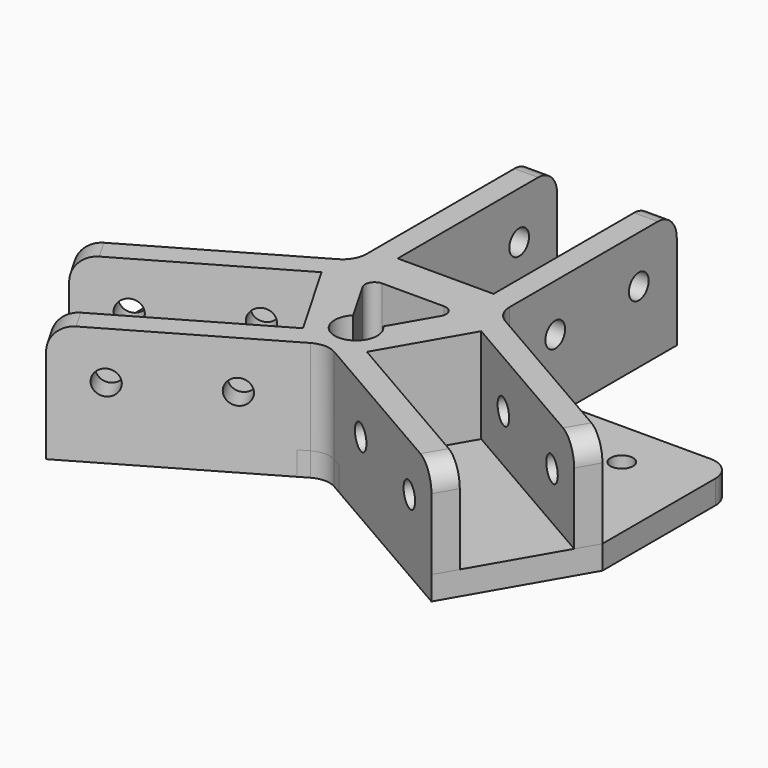
from build123d import *

# Parameters (mm, degrees)
F1_DEPTH    = 20
F2_R        = 2.6
F3_DEPTH    = 50.6016350946
F4_COUNT    = 3
F4_ANGLE    = 240
F6_DEPTH    = 5
F7_T1_DEPTH = 25
F10_DEPTH   = 5
F11_DEPTH   = 25.001
F12_R       = 2
F13_R       = 2.6
F13_R_2     = 2.372590354
F14_DEPTH   = 25.001
F15_R       = 5
F16_R       = 4.5
F17_DEPTH   = 20


# Not quite as in the source:
# - a fillet or chamfer that OpenCascade refuses, or shapes differently, is made with other operations: its cross-section is extruded or revolved along the edge and cut away or added


with BuildPart() as f1:
    # F0 (on Top) → F1 (new body)
    with BuildSketch(Plane.XY):
        Polygon((43.0992290895, -36.5458269543), (6.7261621305, -15.5458269543), (16.8261621305, 1.9478862021), (53.1992290895, -19.0521137979), (55.6992290895, -14.7219867789), (14.8979589003, 8.8346375481), (0, 0), (-0.2020410997, -17.3193296462), (40.5992290895, -40.8759539732), align=None)
    extrude(amount=F1_DEPTH)

    # F2 (on face) → F3 (cut, through all)
    with BuildSketch(Plane(origin=(-7.55, -13.0769835971, 0), x_dir=(0.8660254038, -0.5, 0), z_dir=(-0.5, -0.8660254038, 0))):
        with Locations((45.5979407522, 10)):
            Circle(F2_R)
        with Locations((23.5979407522, 10)):
            Circle(F2_R)
    extrude(amount=-F3_DEPTH, mode=Mode.SUBTRACT)

    # F4: F1 ×3 about axis
    f4_axis = Axis((0, 0, 10), (0, 0, -1))


with BuildPart() as f1_1:
    add(f1.part)
    for i in range(1, F4_COUNT):
        add(f1.part.rotate(f4_axis, i * F4_ANGLE / (F4_COUNT - 1)))

    # F5 (on face) → F6 (join)
    with BuildSketch(Plane(origin=(0, 0, 0), x_dir=(1, 0, 0), z_dir=(0, 0, -1))):
        Polygon((0, 17.4359781295), (-40.5992290895, 40.8759539732), (-55.6992290895, 14.7219867789), (-15.1, -8.7179890648), (-15.1, -55.5979407522), (15.1, -55.5979407522), (15.1, -8.7179890648), (55.6992290895, 14.7219867789), (40.5992290895, 40.8759539732), align=None)
    extrude(amount=F6_DEPTH)

    # F7: fillet of radius 5 on 3 edges, made by hand

    # F7_s2 → F7_t1 (join)
    with BuildSketch(Plane.XY.offset(-5)):
        with BuildLine():
            ThreePointArc((2.5, -18.8792383324), (0, -18.2093653514), (-2.5, -18.8792383324))
            Line((-2.5, -18.8792383324), (-2.55, -18.7926357921))
            ThreePointArc((-2.55, -18.7926357921), (-1.299975, -18.0710489919), (-0.05, -17.3493755891))
            Line((-0.05, -17.3493755891), (0.05, -17.3493755891))
            ThreePointArc((0.05, -17.3493755891), (1.299975, -18.0710489919), (2.55, -18.7926357921))
            Line((2.55, -18.7926357921), (2.5, -18.8792383324))
        make_face()
        with BuildLine():
            ThreePointArc((15.0999, 11.6046826757), (15.7697729811, 9.1046826757), (17.5999, 7.2745556568))
            Line((17.5999, 7.2745556568), (17.5499, 7.1879531164))
            ThreePointArc((17.5499, 7.1879531164), (16.299975, 7.9097131217), (15.05, 8.6313865244))
            Line((15.05, 8.6313865244), (15, 8.7179890648))
            ThreePointArc((15, 8.7179890648), (15, 10.1613358702), (14.9999, 11.6046826757))
            Line((14.9999, 11.6046826757), (15.0999, 11.6046826757))
        make_face()
        with BuildLine():
            ThreePointArc((-17.5999, 7.2745556568), (-15.7697729811, 9.1046826757), (-15.0999, 11.6046826757))
            Line((-15.0999, 11.6046826757), (-14.9999, 11.6046826757))
            ThreePointArc((-14.9999, 11.6046826757), (-15, 10.1613358702), (-15, 8.7179890648))
            Line((-15, 8.7179890648), (-15.05, 8.6313865244))
            ThreePointArc((-15.05, 8.6313865244), (-16.299975, 7.9097131217), (-17.5499, 7.1879531164))
            Line((-17.5499, 7.1879531164), (-17.5999, 7.2745556568))
        make_face()
    extrude(amount=F7_T1_DEPTH)

    # F9 (on face) → F10 (join)
    with BuildSketch(Plane(origin=(0, 0, -5), x_dir=(1, 0, 0), z_dir=(0, 0, -1))):
        with BuildLine():
            Line((-55.6992290895, 14.7219867789), (-55.6992290895, -20))
            Line((-55.6992290895, -20), (55.6992290895, -20))
            Line((55.6992290895, -20), (55.6992290895, 14.7219867789))
            Line((55.6992290895, 14.7219867789), (52.6519667355, 20))
            Line((52.6519667355, 20), (4.4410161514, 20))
            Line((4.4410161514, 20), (2.5, 18.8793538025))
            ThreePointArc((2.5, 18.8793538025), (0, 18.2094808214), (-2.5, 18.8793538025))
            Line((-2.5, 18.8793538025), (-4.4410161514, 20))
            Line((-4.4410161514, 20), (-52.6519667355, 20))
            Line((-52.6519667355, 20), (-55.6992290895, 14.7219867789))
        make_face()
    extrude(amount=-F10_DEPTH)

    # F8 (on face) → F11 (cut, through all)
    with BuildSketch(Plane.XY.offset(20)):
        Polygon((10, 5.0614941438), (-10, 5.0614941438), (0, -12.2590139319), align=None)
    extrude(amount=-F11_DEPTH, mode=Mode.SUBTRACT)

    # F12
    f12_edges = [f1_1.edges().sort_by_distance(p)[0] for p in [
        (10, 5.061494, 7.5),
        (-10, 5.061494, 7.5),
        (0, -12.259014, 7.5),
    ]]
    fillet(f12_edges, radius=F12_R)

    # F13 (on face) → F14 (cut, through all)
    with BuildSketch(Plane(origin=(0, 0, -5), x_dir=(1, 0, 0), z_dir=(0, 0, -1))):
        with Locations((-40, -10)):
            Circle(F13_R)
        with Locations((40, -10)):
            Circle(F13_R_2)
        with Locations((0, 10)):
            Circle(F13_R)
    extrude(amount=-F14_DEPTH, mode=Mode.SUBTRACT)

    # F15
    f15_edges = [f1_1.edges().sort_by_distance(p)[0] for p in [
        (-15.1, 20, -2.5),
        (15.1, 20, -2.5),
        (55.699229, 20, -2.5),
        (-55.699229, 20, -2.5),
        (-12.6, 55.597941, 20),
        (12.6, 55.597941, 20),
        (-54.449229, -16.88705, 20),
        (-41.849229, -38.71089, 20),
        (54.449229, -16.88705, 20),
        (41.849229, -38.71089, 20),
    ]]
    fillet(f15_edges, radius=F15_R)

    # F16 (on face) → F17 (cut)
    with BuildSketch(Plane.XY.offset(20)):
        with Locations((0, -10)):
            Circle(F16_R)
    extrude(amount=-F17_DEPTH, mode=Mode.SUBTRACT)


solid = f1_1.part
